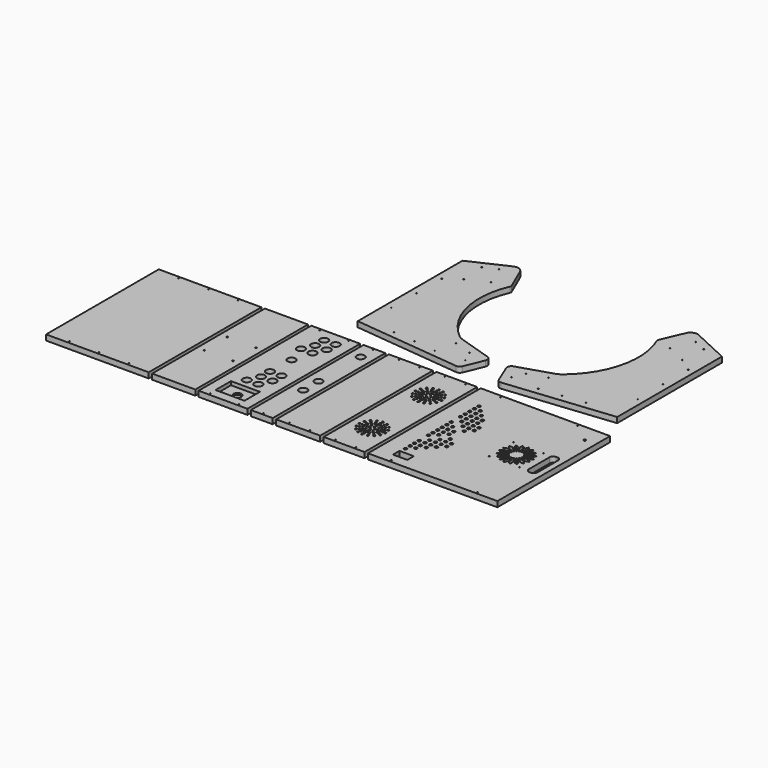
from build123d import *

# Parameters (mm, degrees)
F0_W      = 16
F0_H      = 420.523803
F0_R      = 14
F0_R_2    = 1.6
F1_DEPTH  = 19.05
F2_DEPTH  = 19.05
F0_W_2    = 357
F0_H_2    = 490
F3_DEPTH  = 19.05
F0_R_3    = 2.5
F4_DEPTH  = 19.05
F0_W_3    = 170
F0_W_4    = 98
F0_H_3    = 66
F5_DEPTH  = 19.05
F0_W_5    = 153
F6_DEPTH  = 19.05
F0_W_6    = 76
F7_DEPTH  = 19.05
F0_W_7    = 142
F0_R_4    = 3
F8_DEPTH  = 19.05
F0_W_8    = 450
F0_W_9    = 49.9710738659
F0_H_4    = 28.1445980072
F0_R_5    = 5
F0_R_6    = 1.75
F0_R_7    = 4
F9_DEPTH  = 19.05
F10_W     = 100.751042366
F10_H     = 67.1674013138
F10_R     = 14
F11_DEPTH = 12.7


# Not quite as in the source:
# - ends of sketch curves that miss each other by under 0.0002 mm in the source are joined
# - the dataset's text gives a spline's control points without its knots; the knots are read off the source's solid


with BuildPart() as f1:
    # F0 (on Top) → F1 (new body)
    with BuildSketch(Plane.XY):
        with BuildLine():
            ThreePointArc((118.5482367504, 140.3838887016), (29.2680787824, 284.7869007763), (44.0792440047, 453.913497998))
            ThreePointArc((44.0792440047, 453.913497998), (44.6945754076, 456.8856380721), (44.0816068861, 459.8582663821))
            Line((44.0816068861, 459.8582663821), (10.171633, 538.500267))
            ThreePointArc((10.171633, 538.500267), (-3.8765949653, 551.9603339279), (-23.3202071387, 551.2732802984))
            Line((-23.3202071387, 551.2732802984), (-152.1134, 491.42611))
            Line((-152.1134, 491.42611), (-152.1134, 35.994447))
            Line((-152.1134, 35.994447), (220.668635, -2.682718))
            ThreePointArc((220.668635, -2.682718), (229.9119854484, -0.638415896), (236.0902296243, 6.5343101544))
            Line((236.0902296243, 6.5343101544), (263.285491, 72.693217))
            ThreePointArc((263.285491, 72.693217), (263.0041902378, 84.740313744), (253.9506129321, 92.6929487862))
            Line((253.9506129321, 92.6929487862), (138.885599, 129.221951))
            ThreePointArc((138.885599, 129.221951), (128.172308682, 133.81062664), (118.5482367504, 140.3838887016))
        make_face()
        with Locations((-129.1134, 263.2859435)):
            Rectangle(F0_W, F0_H, mode=Mode.SUBTRACT)
        Polygon((20.257829, 446.91905), (-106.753851, 387.899707), (-113.091563, 402.597754), (13.920117, 461.617097), align=None, mode=Mode.SUBTRACT)
        Polygon((-11.034626, 519.490656), (-112.233483, 472.465925), (-118.975929, 486.975902), (-17.372338, 534.188703), align=None, mode=Mode.SUBTRACT)
        Polygon((196.938753, 31.951096), (195.287572, 16.036524), (-112.166792, 47.935762), (-110.515612, 63.850334), align=None, mode=Mode.SUBTRACT)
        with Locations((174.758149, 57.146597)):
            Circle(F0_R, mode=Mode.SUBTRACT)
        Polygon((96.986505, 104.752845), (103.090393, 119.601996), (241.766108, 75.577446), (235.66222, 60.728295), align=None, mode=Mode.SUBTRACT)
        Polygon((203.468062, 21.862117), (220.744217, 63.89045), (235.0899798126, 59.3361864098), (217.341675, 16.159233), align=None, mode=Mode.SUBTRACT)
        with Locations((-129.1134, 263.2859435)):
            Rectangle(F0_W, F0_H)
        with Locations((-129.6134, 153.285944)):
            Circle(F0_R_2, mode=Mode.SUBTRACT)
        with Locations((-129.6134, 263.285944)):
            Circle(F0_R_2, mode=Mode.SUBTRACT)
        with Locations((-129.6134, 373.285944)):
            Circle(F0_R_2, mode=Mode.SUBTRACT)
        Polygon((-113.091563, 402.597754), (-106.753851, 387.899707), (20.257829, 446.91905), (13.920117, 461.617097), align=None)
        with Locations((-80.973898, 408.376093)):
            Circle(F0_R_2, mode=Mode.SUBTRACT)
        with Locations((-11.54993, 440.408904)):
            Circle(F0_R_2, mode=Mode.SUBTRACT)
        Polygon((-118.975929, 486.975902), (-112.233483, 472.465925), (-11.034626, 519.490656), (-17.372338, 534.188703), align=None)
        with Locations((-87.024666, 493.674259)):
            Circle(F0_R_2, mode=Mode.SUBTRACT)
        with Locations((-43.238492, 513.899138)):
            Circle(F0_R_2, mode=Mode.SUBTRACT)
        Polygon((235.0899798126, 59.3361864098), (220.744217, 63.89045), (203.468062, 21.862117), (217.341675, 16.159233), align=None)
        with Locations((219.042946, 40.024842)):
            Circle(F0_R_2, mode=Mode.SUBTRACT)
        Polygon((241.766108, 75.577446), (103.090393, 119.601996), (96.986505, 104.752845), (235.66222, 60.728295), align=None)
        with Locations((138.165875, 100.597925)):
            Circle(F0_R_2, mode=Mode.SUBTRACT)
        with Locations((200.978281, 80.69215)):
            Circle(F0_R_2, mode=Mode.SUBTRACT)
        with Locations((174.758149, 57.146597)):
            Circle(F0_R)
        Polygon((-112.166792, 47.935762), (195.287572, 16.036524), (196.938753, 31.951096), (-110.515612, 63.850334), align=None)
        with Locations((-34.52921, 47.420908)):
            Circle(F0_R_2, mode=Mode.SUBTRACT)
        with Locations((42.334381, 39.446099)):
            Circle(F0_R_2, mode=Mode.SUBTRACT)
        with Locations((119.215626, 31.64332)):
            Circle(F0_R_2, mode=Mode.SUBTRACT)
    extrude(amount=F1_DEPTH)


with BuildPart() as f2:
    # F0 (on Top) → F2 (new body)
    with BuildSketch(Plane.XY):
        with BuildLine():
            Line((588.126429, 538.500267), (554.216456, 459.858266))
            ThreePointArc((554.216456, 459.858266), (553.6034865924, 456.8856380721), (554.2188179042, 453.9134979586))
            ThreePointArc((554.2188179042, 453.9134979586), (569.0299832176, 284.7869007763), (479.7498252496, 140.3838887016))
            ThreePointArc((479.7498252496, 140.3838887016), (470.125753318, 133.81062664), (459.4124630169, 129.2219509467))
            Line((459.4124630169, 129.2219509467), (344.347449, 92.692949))
            ThreePointArc((344.347449, 92.692949), (335.2938717622, 84.740313744), (335.0125713757, 72.6932171544))
            Line((335.0125713757, 72.6932171544), (362.207832, 6.53431))
            ThreePointArc((362.207832, 6.53431), (368.3860765516, -0.638415896), (377.6294270257, -2.682718248))
            Line((377.6294270257, -2.682718248), (750.411462, 35.994447))
            Line((750.411462, 35.994447), (750.411462, 491.42611))
            Line((750.411462, 491.42611), (621.618269, 551.27328))
            ThreePointArc((621.618269, 551.27328), (602.1746569653, 551.9603339279), (588.126429, 538.500267))
        make_face()
        Polygon((363.2080821874, 59.3361864098), (377.553845, 63.89045), (394.83, 21.862117), (380.956387, 16.159233), align=None, mode=Mode.SUBTRACT)
        with Locations((423.539913, 57.146597)):
            Circle(F0_R, mode=Mode.SUBTRACT)
        Polygon((710.464854, 47.935762), (403.01049, 16.036524), (401.359309, 31.951096), (708.813674, 63.850334), align=None, mode=Mode.SUBTRACT)
        Polygon((356.531954, 75.577446), (495.207669, 119.601996), (501.311557, 104.752845), (362.635842, 60.728295), align=None, mode=Mode.SUBTRACT)
        with Locations((727.411462, 263.2859435)):
            Rectangle(F0_W, F0_H, mode=Mode.SUBTRACT)
        Polygon((711.389625, 402.597754), (705.051913, 387.899707), (578.040233, 446.91905), (584.377945, 461.617097), align=None, mode=Mode.SUBTRACT)
        Polygon((717.273991, 486.975902), (710.531545, 472.465925), (609.332688, 519.490656), (615.6704, 534.188703), align=None, mode=Mode.SUBTRACT)
        Polygon((609.332688, 519.490656), (710.531545, 472.465925), (717.273991, 486.975902), (615.6704, 534.188703), align=None)
        with Locations((641.536554, 513.899138)):
            Circle(F0_R_2, mode=Mode.SUBTRACT)
        with Locations((685.322728, 493.674259)):
            Circle(F0_R_2, mode=Mode.SUBTRACT)
        Polygon((578.040233, 446.91905), (705.051913, 387.899707), (711.389625, 402.597754), (584.377945, 461.617097), align=None)
        with Locations((679.27196, 408.376093)):
            Circle(F0_R_2, mode=Mode.SUBTRACT)
        with Locations((609.847992, 440.408904)):
            Circle(F0_R_2, mode=Mode.SUBTRACT)
        with Locations((727.411462, 263.2859435)):
            Rectangle(F0_W, F0_H)
        with Locations((727.911462, 153.285944)):
            Circle(F0_R_2, mode=Mode.SUBTRACT)
        with Locations((727.911462, 263.285944)):
            Circle(F0_R_2, mode=Mode.SUBTRACT)
        with Locations((727.911462, 373.285944)):
            Circle(F0_R_2, mode=Mode.SUBTRACT)
        Polygon((501.311557, 104.752845), (495.207669, 119.601996), (356.531954, 75.577446), (362.635842, 60.728295), align=None)
        with Locations((397.319781, 80.69215)):
            Circle(F0_R_2, mode=Mode.SUBTRACT)
        with Locations((460.132187, 100.597925)):
            Circle(F0_R_2, mode=Mode.SUBTRACT)
        with Locations((423.539913, 57.146597)):
            Circle(F0_R)
        Polygon((394.83, 21.862117), (377.553845, 63.89045), (363.2080821874, 59.3361864098), (380.956387, 16.159233), align=None)
        with Locations((379.255116, 40.024842)):
            Circle(F0_R_2, mode=Mode.SUBTRACT)
        Polygon((401.359309, 31.951096), (403.01049, 16.036524), (710.464854, 47.935762), (708.813674, 63.850334), align=None)
        with Locations((479.082436, 31.64332)):
            Circle(F0_R_2, mode=Mode.SUBTRACT)
        with Locations((555.963681, 39.446099)):
            Circle(F0_R_2, mode=Mode.SUBTRACT)
        with Locations((632.827272, 47.420908)):
            Circle(F0_R_2, mode=Mode.SUBTRACT)
    extrude(amount=F2_DEPTH)


with BuildPart() as f3:
    # F0 (on Top) → F3 (new body)
    with BuildSketch(Plane.XY):
        with Locations((-586.06424, -308.60144)):
            Rectangle(F0_W_2, F0_H_2)
        with Locations((-689.56424, -546.10144)):
            Circle(F0_R_2, mode=Mode.SUBTRACT)
        with Locations((-586.06424, -546.10144)):
            Circle(F0_R_2, mode=Mode.SUBTRACT)
        with Locations((-482.56424, -546.10144)):
            Circle(F0_R_2, mode=Mode.SUBTRACT)
        with Locations((-689.56424, -71.10144)):
            Circle(F0_R_2, mode=Mode.SUBTRACT)
        with Locations((-586.06424, -71.10144)):
            Circle(F0_R_2, mode=Mode.SUBTRACT)
        with Locations((-482.56424, -71.10144)):
            Circle(F0_R_2, mode=Mode.SUBTRACT)
    extrude(amount=F3_DEPTH)


with BuildPart() as f4:
    # F0 (on Top) → F4 (new body)
    with BuildSketch(Plane.XY):
        Polygon((-395.373191, -518.60144), (-395.373191, -533.60144), (-395.373191, -553.60144), (-245.373191, -553.60144), (-245.373191, -533.60144), (-245.373191, -518.60144), (-245.373191, -98.60144), (-245.373191, -83.60144), (-245.373191, -63.60144), (-395.373191, -63.60144), align=None)
        with Locations((-370.373191, -358.60144)):
            Circle(F0_R_3, mode=Mode.SUBTRACT)
        with Locations((-270.373191, -358.60144)):
            Circle(F0_R_3, mode=Mode.SUBTRACT)
        with Locations((-370.373191, -258.60144)):
            Circle(F0_R_3, mode=Mode.SUBTRACT)
        with Locations((-270.373191, -258.60144)):
            Circle(F0_R_3, mode=Mode.SUBTRACT)
    extrude(amount=F4_DEPTH)


with BuildPart() as f5:
    # F0 (on Top) → F5 (new body)
    with BuildSketch(Plane.XY):
        with Locations((-149.025639, -308.60144)):
            Rectangle(F0_W_3, F0_H_2)
        with Locations((-199.025639, -546.60144)):
            Circle(F0_R_2, mode=Mode.SUBTRACT)
        with Locations((-99.025639, -546.60144)):
            Circle(F0_R_2, mode=Mode.SUBTRACT)
        with Locations((-150.025639, -489.60144)):
            Rectangle(F0_W_4, F0_H_3, mode=Mode.SUBTRACT)
        with Locations((-171.025639, -422.60144)):
            Circle(F0_R, mode=Mode.SUBTRACT)
        with Locations((-131.025639, -422.60144)):
            Circle(F0_R, mode=Mode.SUBTRACT)
        with Locations((-153.025639, -383.35144)):
            Circle(F0_R, mode=Mode.SUBTRACT)
        with Locations((-113.025639, -383.35144)):
            Circle(F0_R, mode=Mode.SUBTRACT)
        with Locations((-153.025639, -344.10144)):
            Circle(F0_R, mode=Mode.SUBTRACT)
        with Locations((-113.025639, -344.10144)):
            Circle(F0_R, mode=Mode.SUBTRACT)
        with Locations((-150.025639, -254.35144)):
            Rectangle(F0_W_4, F0_H_3, mode=Mode.SUBTRACT)
        with Locations((-171.025639, -187.35144)):
            Circle(F0_R, mode=Mode.SUBTRACT)
        with Locations((-131.025639, -187.35144)):
            Circle(F0_R, mode=Mode.SUBTRACT)
        with Locations((-153.025639, -148.10144)):
            Circle(F0_R, mode=Mode.SUBTRACT)
        with Locations((-113.025639, -148.10144)):
            Circle(F0_R, mode=Mode.SUBTRACT)
        with Locations((-199.025639, -70.60144)):
            Circle(F0_R_2, mode=Mode.SUBTRACT)
        with Locations((-153.025639, -108.85144)):
            Circle(F0_R, mode=Mode.SUBTRACT)
        with Locations((-113.025639, -108.85144)):
            Circle(F0_R, mode=Mode.SUBTRACT)
        with Locations((-99.025639, -70.60144)):
            Circle(F0_R_2, mode=Mode.SUBTRACT)
        with Locations((-150.025639, -254.35144)):
            Rectangle(F0_W_4, F0_H_3)
        with Locations((-150.025639, -254.35144)):
            Circle(F0_R, mode=Mode.SUBTRACT)
        with Locations((-150.025639, -489.60144)):
            Rectangle(F0_W_4, F0_H_3)
        with Locations((-150.025639, -489.60144)):
            Circle(F0_R, mode=Mode.SUBTRACT)
    extrude(amount=F5_DEPTH)

    # F10 (on face) → F11 (cut)
    with BuildSketch(Plane.XY.offset(19.05)):
        with Locations((-150.2750962973, -488.087952137)):
            Rectangle(F10_W, F10_H)
        with Locations((-150.025639, -489.60144)):
            Circle(F10_R, mode=Mode.SUBTRACT)
    extrude(amount=-F11_DEPTH, mode=Mode.SUBTRACT)


with BuildPart() as f6:
    # F0 (on Top) → F6 (new body)
    with BuildSketch(Plane.XY):
        with Locations((112.484238, -308.60144)):
            Rectangle(F0_W_5, F0_H_2)
        with Locations((76.484238, -546.60144)):
            Circle(F0_R_2, mode=Mode.SUBTRACT)
        with Locations((148.484238, -546.60144)):
            Circle(F0_R_2, mode=Mode.SUBTRACT)
        with Locations((76.484238, -70.60144)):
            Circle(F0_R_2, mode=Mode.SUBTRACT)
        with Locations((148.484238, -70.60144)):
            Circle(F0_R_2, mode=Mode.SUBTRACT)
    extrude(amount=F6_DEPTH)


with BuildPart() as f7:
    # F0 (on Top) → F7 (new body)
    with BuildSketch(Plane.XY):
        with Locations((-14.20681, -308.60144)):
            Rectangle(F0_W_6, F0_H_2)
        with Locations((-14.20681, -546.60144)):
            Circle(F0_R_2, mode=Mode.SUBTRACT)
        with Locations((-14.20681, -373.60144)):
            Circle(F0_R, mode=Mode.SUBTRACT)
        with Locations((-14.20681, -306.99525)):
            Circle(F0_R, mode=Mode.SUBTRACT)
        with Locations((-14.20681, -123.560914)):
            Circle(F0_R, mode=Mode.SUBTRACT)
        with Locations((-14.20681, -70.60144)):
            Circle(F0_R_2, mode=Mode.SUBTRACT)
    extrude(amount=F7_DEPTH)


with BuildPart() as f8:
    # F0 (on Top) → F8 (new body)
    with BuildSketch(Plane.XY):
        with Locations((272.175287, -308.60144)):
            Rectangle(F0_W_7, F0_H_2)
        with Locations((236.175287, -546.60144)):
            Circle(F0_R_2, mode=Mode.SUBTRACT)
        with Locations((308.175287, -546.60144)):
            Circle(F0_R_2, mode=Mode.SUBTRACT)
        with Locations((254.954532, -472.176019)):
            Circle(F0_R_4, mode=Mode.SUBTRACT)
        with Locations((240.355481, -462.421245)):
            Circle(F0_R_4, mode=Mode.SUBTRACT)
        with Locations((258.398683, -463.861103)):
            Circle(F0_R_4, mode=Mode.SUBTRACT)
        with Locations((246.719442, -456.057284)):
            Circle(F0_R_4, mode=Mode.SUBTRACT)
        with Locations((261.842834, -455.546188)):
            Circle(F0_R_4, mode=Mode.SUBTRACT)
        with Locations((272.175287, -475.60144)):
            Circle(F0_R_4, mode=Mode.SUBTRACT)
        with Locations((289.396041, -472.176019)):
            Circle(F0_R_4, mode=Mode.SUBTRACT)
        with Locations((272.175287, -466.60144)):
            Circle(F0_R_4, mode=Mode.SUBTRACT)
        with Locations((285.95189, -463.861103)):
            Circle(F0_R_4, mode=Mode.SUBTRACT)
        with Locations((272.175287, -457.60144)):
            Circle(F0_R_4, mode=Mode.SUBTRACT)
        with Locations((282.507739, -455.546188)):
            Circle(F0_R_4, mode=Mode.SUBTRACT)
        with Locations((303.995092, -462.421245)):
            Circle(F0_R_4, mode=Mode.SUBTRACT)
        with Locations((297.631131, -456.057284)):
            Circle(F0_R_4, mode=Mode.SUBTRACT)
        with Locations((230.600708, -447.822195)):
            Circle(F0_R_4, mode=Mode.SUBTRACT)
        with Locations((238.915623, -444.378044)):
            Circle(F0_R_4, mode=Mode.SUBTRACT)
        with Locations((253.083403, -449.693323)):
            Circle(F0_R_4, mode=Mode.SUBTRACT)
        with Locations((259.447364, -443.329362)):
            Circle(F0_R_4, mode=Mode.SUBTRACT)
        with Locations((247.230539, -440.933893)):
            Circle(F0_R_4, mode=Mode.SUBTRACT)
        with Locations((227.175287, -430.60144)):
            Circle(F0_R_4, mode=Mode.SUBTRACT)
        with Locations((236.175287, -430.60144)):
            Circle(F0_R_4, mode=Mode.SUBTRACT)
        with Locations((238.915623, -416.824837)):
            Circle(F0_R_4, mode=Mode.SUBTRACT)
        with Locations((245.175287, -430.60144)):
            Circle(F0_R_4, mode=Mode.SUBTRACT)
        with Locations((254.175287, -430.60144)):
            Circle(F0_R_4, mode=Mode.SUBTRACT)
        with Locations((263.175287, -430.60144)):
            Circle(F0_R_4, mode=Mode.SUBTRACT)
        with Locations((247.230539, -420.268988)):
            Circle(F0_R_4, mode=Mode.SUBTRACT)
        with Locations((259.447364, -417.873518)):
            Circle(F0_R_4, mode=Mode.SUBTRACT)
        with Locations((272.175287, -448.60144)):
            Circle(F0_R_4, mode=Mode.SUBTRACT)
        with Locations((284.903209, -443.329362)):
            Circle(F0_R_4, mode=Mode.SUBTRACT)
        with Locations((272.175287, -439.60144)):
            Circle(F0_R_4, mode=Mode.SUBTRACT)
        with Locations((291.26717, -449.693323)):
            Circle(F0_R_4, mode=Mode.SUBTRACT)
        with Locations((313.749866, -447.822195)):
            Circle(F0_R_4, mode=Mode.SUBTRACT)
        with Locations((305.43495, -444.378044)):
            Circle(F0_R_4, mode=Mode.SUBTRACT)
        with Locations((297.120034, -440.933893)):
            Circle(F0_R_4, mode=Mode.SUBTRACT)
        with Locations((281.175287, -430.60144)):
            Circle(F0_R_4, mode=Mode.SUBTRACT)
        with Locations((290.175287, -430.60144)):
            Circle(F0_R_4, mode=Mode.SUBTRACT)
        with Locations((272.175287, -421.60144)):
            Circle(F0_R_4, mode=Mode.SUBTRACT)
        with Locations((284.903209, -417.873518)):
            Circle(F0_R_4, mode=Mode.SUBTRACT)
        with Locations((299.175287, -430.60144)):
            Circle(F0_R_4, mode=Mode.SUBTRACT)
        with Locations((308.175287, -430.60144)):
            Circle(F0_R_4, mode=Mode.SUBTRACT)
        with Locations((297.120034, -420.268988)):
            Circle(F0_R_4, mode=Mode.SUBTRACT)
        with Locations((305.43495, -416.824837)):
            Circle(F0_R_4, mode=Mode.SUBTRACT)
        with Locations((317.175287, -430.60144)):
            Circle(F0_R_4, mode=Mode.SUBTRACT)
        with Locations((230.600708, -413.380686)):
            Circle(F0_R_4, mode=Mode.SUBTRACT)
        with Locations((240.355481, -398.781635)):
            Circle(F0_R_4, mode=Mode.SUBTRACT)
        with Locations((253.083403, -411.509557)):
            Circle(F0_R_4, mode=Mode.SUBTRACT)
        with Locations((246.719442, -405.145596)):
            Circle(F0_R_4, mode=Mode.SUBTRACT)
        with Locations((261.842834, -405.656693)):
            Circle(F0_R_4, mode=Mode.SUBTRACT)
        with Locations((258.398683, -397.341777)):
            Circle(F0_R_4, mode=Mode.SUBTRACT)
        with Locations((254.954532, -389.026861)):
            Circle(F0_R_4, mode=Mode.SUBTRACT)
        with Locations((272.175287, -412.60144)):
            Circle(F0_R_4, mode=Mode.SUBTRACT)
        with Locations((272.175287, -403.60144)):
            Circle(F0_R_4, mode=Mode.SUBTRACT)
        with Locations((282.507739, -405.656693)):
            Circle(F0_R_4, mode=Mode.SUBTRACT)
        with Locations((291.26717, -411.509557)):
            Circle(F0_R_4, mode=Mode.SUBTRACT)
        with Locations((313.749866, -413.380686)):
            Circle(F0_R_4, mode=Mode.SUBTRACT)
        with Locations((297.631131, -405.145596)):
            Circle(F0_R_4, mode=Mode.SUBTRACT)
        with Locations((303.995092, -398.781635)):
            Circle(F0_R_4, mode=Mode.SUBTRACT)
        with Locations((272.175287, -394.60144)):
            Circle(F0_R_4, mode=Mode.SUBTRACT)
        with Locations((285.95189, -397.341777)):
            Circle(F0_R_4, mode=Mode.SUBTRACT)
        with Locations((272.175287, -385.60144)):
            Circle(F0_R_4, mode=Mode.SUBTRACT)
        with Locations((289.396041, -389.026861)):
            Circle(F0_R_4, mode=Mode.SUBTRACT)
        with Locations((254.954532, -228.176019)):
            Circle(F0_R_4, mode=Mode.SUBTRACT)
        with Locations((240.355481, -218.421245)):
            Circle(F0_R_4, mode=Mode.SUBTRACT)
        with Locations((258.398683, -219.861103)):
            Circle(F0_R_4, mode=Mode.SUBTRACT)
        with Locations((246.719442, -212.057284)):
            Circle(F0_R_4, mode=Mode.SUBTRACT)
        with Locations((261.842834, -211.546188)):
            Circle(F0_R_4, mode=Mode.SUBTRACT)
        with Locations((272.175287, -231.60144)):
            Circle(F0_R_4, mode=Mode.SUBTRACT)
        with Locations((289.396041, -228.176019)):
            Circle(F0_R_4, mode=Mode.SUBTRACT)
        with Locations((272.175287, -222.60144)):
            Circle(F0_R_4, mode=Mode.SUBTRACT)
        with Locations((285.95189, -219.861103)):
            Circle(F0_R_4, mode=Mode.SUBTRACT)
        with Locations((272.175287, -213.60144)):
            Circle(F0_R_4, mode=Mode.SUBTRACT)
        with Locations((282.507739, -211.546188)):
            Circle(F0_R_4, mode=Mode.SUBTRACT)
        with Locations((303.995092, -218.421245)):
            Circle(F0_R_4, mode=Mode.SUBTRACT)
        with Locations((297.631131, -212.057284)):
            Circle(F0_R_4, mode=Mode.SUBTRACT)
        with Locations((230.600708, -203.822195)):
            Circle(F0_R_4, mode=Mode.SUBTRACT)
        with Locations((238.915623, -200.378044)):
            Circle(F0_R_4, mode=Mode.SUBTRACT)
        with Locations((253.083403, -205.693323)):
            Circle(F0_R_4, mode=Mode.SUBTRACT)
        with Locations((259.447364, -199.329362)):
            Circle(F0_R_4, mode=Mode.SUBTRACT)
        with Locations((247.230539, -196.933893)):
            Circle(F0_R_4, mode=Mode.SUBTRACT)
        with Locations((227.175287, -186.60144)):
            Circle(F0_R_4, mode=Mode.SUBTRACT)
        with Locations((236.175287, -186.60144)):
            Circle(F0_R_4, mode=Mode.SUBTRACT)
        with Locations((245.175287, -186.60144)):
            Circle(F0_R_4, mode=Mode.SUBTRACT)
        with Locations((254.175287, -186.60144)):
            Circle(F0_R_4, mode=Mode.SUBTRACT)
        with Locations((263.175287, -186.60144)):
            Circle(F0_R_4, mode=Mode.SUBTRACT)
        with Locations((247.230539, -176.268988)):
            Circle(F0_R_4, mode=Mode.SUBTRACT)
        with Locations((259.447364, -173.873518)):
            Circle(F0_R_4, mode=Mode.SUBTRACT)
        with Locations((272.175287, -204.60144)):
            Circle(F0_R_4, mode=Mode.SUBTRACT)
        with Locations((284.903209, -199.329362)):
            Circle(F0_R_4, mode=Mode.SUBTRACT)
        with Locations((272.175287, -195.60144)):
            Circle(F0_R_4, mode=Mode.SUBTRACT)
        with Locations((291.26717, -205.693323)):
            Circle(F0_R_4, mode=Mode.SUBTRACT)
        with Locations((313.749866, -203.822195)):
            Circle(F0_R_4, mode=Mode.SUBTRACT)
        with Locations((305.43495, -200.378044)):
            Circle(F0_R_4, mode=Mode.SUBTRACT)
        with Locations((297.120034, -196.933893)):
            Circle(F0_R_4, mode=Mode.SUBTRACT)
        with Locations((281.175287, -186.60144)):
            Circle(F0_R_4, mode=Mode.SUBTRACT)
        with Locations((290.175287, -186.60144)):
            Circle(F0_R_4, mode=Mode.SUBTRACT)
        with Locations((272.175287, -177.60144)):
            Circle(F0_R_4, mode=Mode.SUBTRACT)
        with Locations((284.903209, -173.873518)):
            Circle(F0_R_4, mode=Mode.SUBTRACT)
        with Locations((299.175287, -186.60144)):
            Circle(F0_R_4, mode=Mode.SUBTRACT)
        with Locations((308.175287, -186.60144)):
            Circle(F0_R_4, mode=Mode.SUBTRACT)
        with Locations((297.120034, -176.268988)):
            Circle(F0_R_4, mode=Mode.SUBTRACT)
        with Locations((230.600708, -169.380686)):
            Circle(F0_R_4, mode=Mode.SUBTRACT)
        with Locations((238.915623, -172.824837)):
            Circle(F0_R_4, mode=Mode.SUBTRACT)
        with Locations((253.083403, -167.509557)):
            Circle(F0_R_4, mode=Mode.SUBTRACT)
        with Locations((246.719442, -161.145596)):
            Circle(F0_R_4, mode=Mode.SUBTRACT)
        with Locations((261.842834, -161.656693)):
            Circle(F0_R_4, mode=Mode.SUBTRACT)
        with Locations((240.355481, -154.781635)):
            Circle(F0_R_4, mode=Mode.SUBTRACT)
        with Locations((258.398683, -153.341777)):
            Circle(F0_R_4, mode=Mode.SUBTRACT)
        with Locations((254.954532, -145.026861)):
            Circle(F0_R_4, mode=Mode.SUBTRACT)
        with Locations((272.175287, -168.60144)):
            Circle(F0_R_4, mode=Mode.SUBTRACT)
        with Locations((272.175287, -159.60144)):
            Circle(F0_R_4, mode=Mode.SUBTRACT)
        with Locations((282.507739, -161.656693)):
            Circle(F0_R_4, mode=Mode.SUBTRACT)
        with Locations((291.26717, -167.509557)):
            Circle(F0_R_4, mode=Mode.SUBTRACT)
        with Locations((305.43495, -172.824837)):
            Circle(F0_R_4, mode=Mode.SUBTRACT)
        with Locations((313.749866, -169.380686)):
            Circle(F0_R_4, mode=Mode.SUBTRACT)
        with Locations((297.631131, -161.145596)):
            Circle(F0_R_4, mode=Mode.SUBTRACT)
        with Locations((272.175287, -150.60144)):
            Circle(F0_R_4, mode=Mode.SUBTRACT)
        with Locations((285.95189, -153.341777)):
            Circle(F0_R_4, mode=Mode.SUBTRACT)
        with Locations((272.175287, -141.60144)):
            Circle(F0_R_4, mode=Mode.SUBTRACT)
        with Locations((289.396041, -145.026861)):
            Circle(F0_R_4, mode=Mode.SUBTRACT)
        with Locations((303.995092, -154.781635)):
            Circle(F0_R_4, mode=Mode.SUBTRACT)
        with Locations((317.175287, -186.60144)):
            Circle(F0_R_4, mode=Mode.SUBTRACT)
        with Locations((236.175287, -70.60144)):
            Circle(F0_R_2, mode=Mode.SUBTRACT)
        with Locations((308.175287, -70.60144)):
            Circle(F0_R_2, mode=Mode.SUBTRACT)
    extrude(amount=F8_DEPTH)


with BuildPart() as f9:
    # F0 (on Top) → F9 (new body)
    with BuildSketch(Plane.XY):
        with Locations((580.366335, -308.60144)):
            Rectangle(F0_W_8, F0_H_2)
        with Locations((430.366335, -546.10144)):
            Circle(F0_R_2, mode=Mode.SUBTRACT)
        with Locations((438.1191283464, -503.1597018242)):
            Rectangle(F0_W_9, F0_H_4, mode=Mode.SUBTRACT)
        with Locations((417.50945, -468.60144)):
            Circle(F0_R_5, mode=Mode.SUBTRACT)
        with Locations((417.50945, -448.60144)):
            Circle(F0_R_5, mode=Mode.SUBTRACT)
        with Locations((437.50945, -448.60144)):
            Circle(F0_R_5, mode=Mode.SUBTRACT)
        with Locations((417.50945, -428.60144)):
            Circle(F0_R_5, mode=Mode.SUBTRACT)
        with Locations((437.50945, -428.60144)):
            Circle(F0_R_5, mode=Mode.SUBTRACT)
        with Locations((457.50945, -428.60144)):
            Circle(F0_R_5, mode=Mode.SUBTRACT)
        with Locations((730.366335, -546.10144)):
            Circle(F0_R_2, mode=Mode.SUBTRACT)
        with Locations((417.50945, -408.60144)):
            Circle(F0_R_5, mode=Mode.SUBTRACT)
        with Locations((437.50945, -408.60144)):
            Circle(F0_R_5, mode=Mode.SUBTRACT)
        with Locations((457.50945, -408.60144)):
            Circle(F0_R_5, mode=Mode.SUBTRACT)
        with Locations((437.50945, -388.60144)):
            Circle(F0_R_5, mode=Mode.SUBTRACT)
        with Locations((457.50945, -388.60144)):
            Circle(F0_R_5, mode=Mode.SUBTRACT)
        with Locations((477.50945, -408.60144)):
            Circle(F0_R_5, mode=Mode.SUBTRACT)
        with Locations((477.50945, -388.60144)):
            Circle(F0_R_5, mode=Mode.SUBTRACT)
        with Locations((497.50945, -388.60144)):
            Circle(F0_R_5, mode=Mode.SUBTRACT)
        with Locations((417.50945, -368.60144)):
            Circle(F0_R_5, mode=Mode.SUBTRACT)
        with Locations((457.50945, -368.60144)):
            Circle(F0_R_5, mode=Mode.SUBTRACT)
        with Locations((417.50945, -348.60144)):
            Circle(F0_R_5, mode=Mode.SUBTRACT)
        with Locations((437.50945, -348.60144)):
            Circle(F0_R_5, mode=Mode.SUBTRACT)
        with Locations((477.50945, -368.60144)):
            Circle(F0_R_5, mode=Mode.SUBTRACT)
        with Locations((497.50945, -368.60144)):
            Circle(F0_R_5, mode=Mode.SUBTRACT)
        with Locations((477.50945, -348.60144)):
            Circle(F0_R_5, mode=Mode.SUBTRACT)
        with Locations((417.50945, -328.60144)):
            Circle(F0_R_5, mode=Mode.SUBTRACT)
        with Locations((437.50945, -328.60144)):
            Circle(F0_R_5, mode=Mode.SUBTRACT)
        with Locations((457.50945, -328.60144)):
            Circle(F0_R_5, mode=Mode.SUBTRACT)
        with Locations((417.50945, -308.60144)):
            Circle(F0_R_5, mode=Mode.SUBTRACT)
        with Locations((437.50945, -308.60144)):
            Circle(F0_R_5, mode=Mode.SUBTRACT)
        with Locations((457.50945, -308.60144)):
            Circle(F0_R_5, mode=Mode.SUBTRACT)
        with Locations((417.50945, -288.60144)):
            Circle(F0_R_5, mode=Mode.SUBTRACT)
        with Locations((437.50945, -288.60144)):
            Circle(F0_R_5, mode=Mode.SUBTRACT)
        with Locations((477.50945, -288.60144)):
            Circle(F0_R_5, mode=Mode.SUBTRACT)
        with Locations((623.107999, -361.10144)):
            Circle(F0_R_6, mode=Mode.SUBTRACT)
        with Locations((728.107999, -361.10144)):
            Circle(F0_R_6, mode=Mode.SUBTRACT)
        with BuildLine():
            add(Edge.make_bspline(
                [(661.9953345663, -323.6310243721), (662.2030436822, -323.6760680767), (664.8658202707, -324.6021810604), (656.014578, -335.388698), (653.296445, -345.742326), (644.42536, -349.015733), (640.039488, -350.634108)],
                knots=[37.385436, 37.385436, 37.385436, 37.385436, 38.16553, 48.738332, 61.900361, 74.770872, 74.770872, 74.770872, 74.770872], degree=3))
            add(Edge.make_bspline(
                [(640.039488, -350.634108), (640.014511, -346.232188), (639.95701, -336.098186), (653.509426, -332.830412), (655.8785976685, -324.3462786702), (660.5741339851, -323.3228234589), (661.9953345663, -323.6310243721)],
                knots=[0, 0, 0, 0, 12.01872, 27.669227, 32.047827, 37.385436, 37.385436, 37.385436, 37.385436], degree=3))
        make_face(mode=Mode.SUBTRACT)
        with BuildLine():
            add(Edge.make_bspline(
                [(657.6758589757, -318.0688243557), (657.8556358402, -318.1821923098), (660.041077992, -319.963177284), (648.034425, -327.071884), (641.939066, -335.871455), (632.483401, -335.913362), (627.808512, -335.934081)],
                knots=[37.385436, 37.385436, 37.385436, 37.385436, 38.16553, 48.738332, 61.900361, 74.770872, 74.770872, 74.770872, 74.770872], degree=3))
            add(Edge.make_bspline(
                [(627.808512, -335.934081), (629.290587, -331.789087), (632.702587, -322.246573), (646.555337, -323.811069), (651.6833751837, -316.648895877), (656.4457782291, -317.2931308976), (657.6758589757, -318.0688243557)],
                knots=[0, 0, 0, 0, 12.01872, 27.669227, 32.047827, 37.385436, 37.385436, 37.385436, 37.385436], degree=3))
        make_face(mode=Mode.SUBTRACT)
        with BuildLine():
            add(Edge.make_bspline(
                [(655.5192629717, -311.3647179179), (655.6494238634, -311.5327362358), (657.0939353029, -313.9537796275), (643.380051, -316.527262), (634.642656, -322.711419), (625.742905, -319.516771), (621.34286, -317.937334)],
                knots=[37.385436, 37.385436, 37.385436, 37.385436, 38.16553, 48.738332, 61.900361, 74.770872, 74.770872, 74.770872, 74.770872], degree=3))
            add(Edge.make_bspline(
                [(621.34286, -317.937334), (624.153227, -314.549213), (630.62319, -306.749156), (643.105427, -312.957221), (650.3738137707, -307.9808719712), (654.6286678035, -310.21509225), (655.5192629717, -311.3647179179)],
                knots=[0, 0, 0, 0, 12.01872, 27.669227, 32.047827, 37.385436, 37.385436, 37.385436, 37.385436], degree=3))
        make_face(mode=Mode.SUBTRACT)
        with BuildLine():
            add(Edge.make_bspline(
                [(667.9566993628, -327.3804345901), (668.1672879531, -327.3517211294), (670.9862289376, -327.311259493), (666.357988, -340.474573), (667.344928, -351.133457), (660.128406, -357.243543), (656.560551, -360.264375)],
                knots=[37.385436, 37.385436, 37.385436, 37.385436, 38.16553, 48.738332, 61.900361, 74.770872, 74.770872, 74.770872, 74.770872], degree=3))
            add(Edge.make_bspline(
                [(656.560551, -360.264375), (655.031535, -356.136466), (651.511469, -346.633286), (663.12893, -338.927383), (662.4534779475, -330.144600914), (666.5157966577, -327.5768996647), (667.9566993628, -327.3804345901)],
                knots=[0, 0, 0, 0, 12.01872, 27.669227, 32.047827, 37.385436, 37.385436, 37.385436, 37.385436], degree=3))
        make_face(mode=Mode.SUBTRACT)
        with BuildLine():
            add(Edge.make_bspline(
                [(674.8409233367, -328.8648210275), (675.02899128, -328.7658136803), (677.6640903625, -327.7636578564), (677.817085, -341.716078), (682.390058, -351.394599), (677.698518, -359.604398), (675.379017, -363.66333)],
                knots=[37.385436, 37.385436, 37.385436, 37.385436, 38.16553, 48.738332, 61.900361, 74.770872, 74.770872, 74.770872, 74.770872], degree=3))
            add(Edge.make_bspline(
                [(675.379017, -363.66333), (672.530384, -360.307318), (665.972325, -352.581183), (674.253593, -341.366598), (670.61498779, -333.344499859), (673.554112841, -329.542255423), (674.8409233367, -328.8648210275)],
                knots=[0, 0, 0, 0, 12.01872, 27.669227, 32.047827, 37.385436, 37.385436, 37.385436, 37.385436], degree=3))
        make_face(mode=Mode.SUBTRACT)
        with BuildLine():
            add(Edge.make_bspline(
                [(681.8176685037, -327.9051449566), (681.9605320608, -327.7477854641), (684.093957812, -325.904810145), (689.009734, -338.963469), (696.617172, -346.494255), (695.016484, -355.813544), (694.225102, -360.421008)],
                knots=[37.385436, 37.385436, 37.385436, 37.385436, 38.16553, 48.738332, 61.900361, 74.770872, 74.770872, 74.770872, 74.770872], degree=3))
            add(Edge.make_bspline(
                [(694.225102, -360.421008), (690.400439, -358.241679), (681.595385, -353.224475), (685.541618, -339.853851), (679.3787282548, -333.5600210155), (680.8401583471, -328.9818401281), (681.8176685037, -327.9051449566)],
                knots=[0, 0, 0, 0, 12.01872, 27.669227, 32.047827, 37.385436, 37.385436, 37.385436, 37.385436], degree=3))
        make_face(mode=Mode.SUBTRACT)
        with BuildLine():
            add(Edge.make_bspline(
                [(688.0454353909, -324.6171566724), (688.1258630897, -324.4204248936), (689.5002926346, -321.9589198656), (698.585936, -332.548751), (708.31027, -337.023478), (709.993499, -346.328213), (710.825689, -350.928482)],
                knots=[37.385436, 37.385436, 37.385436, 37.385436, 38.16553, 48.738332, 61.900361, 74.770872, 74.770872, 74.770872, 74.770872], degree=3))
            add(Edge.make_bspline(
                [(710.825689, -350.928482), (706.486307, -350.188693), (696.496278, -348.48557), (695.631501, -334.571603), (687.6876631469, -330.7651689726), (687.495127852, -325.963247417), (688.0454353909, -324.6171566724)],
                knots=[0, 0, 0, 0, 12.01872, 27.669227, 32.047827, 37.385436, 37.385436, 37.385436, 37.385436], degree=3))
        make_face(mode=Mode.SUBTRACT)
        with BuildLine():
            add(Edge.make_bspline(
                [(655.7856650626, -304.3273199728), (655.8505106214, -304.5297231889), (656.3798614587, -307.2988117366), (642.612843, -305.026669), (632.287272, -307.849511), (625.016875, -301.803629), (621.422385, -298.81454)],
                knots=[37.385436, 37.385436, 37.385436, 37.385436, 38.16553, 48.738332, 61.900361, 74.770872, 74.770872, 74.770872, 74.770872], degree=3))
            add(Edge.make_bspline(
                [(621.422385, -298.81454), (625.222071, -296.59195), (633.969624, -291.475152), (643.575807, -301.578001), (652.1078684137, -299.3876976547), (655.3419746379, -302.9424237577), (655.7856650626, -304.3273199728)],
                knots=[0, 0, 0, 0, 12.01872, 27.669227, 32.047827, 37.385436, 37.385436, 37.385436, 37.385436], degree=3))
        make_face(mode=Mode.SUBTRACT)
        with BuildLine():
            add(Edge.make_bspline(
                [(658.442933639, -297.8054433781), (658.4346425602, -298.0178186867), (657.9849856295, -300.8009596065), (645.825338, -293.957247), (635.157006, -293.078297), (630.392882, -284.910404), (628.037494, -280.872191)],
                knots=[37.385436, 37.385436, 37.385436, 37.385436, 38.16553, 48.738332, 61.900361, 74.770872, 74.770872, 74.770872, 74.770872], degree=3))
            add(Edge.make_bspline(
                [(628.037494, -280.872191), (632.368202, -280.083209), (642.338261, -278.26683), (647.909742, -291.045911), (656.6763853938, -291.905836018), (658.4996633881, -296.3523154746), (658.442933639, -297.8054433781)],
                knots=[0, 0, 0, 0, 12.01872, 27.669227, 32.047827, 37.385436, 37.385436, 37.385436, 37.385436], degree=3))
        make_face(mode=Mode.SUBTRACT)
        with BuildLine():
            add(Edge.make_bspline(
                [(663.1705620516, -292.5857233777), (663.090134334, -292.7824551636), (661.7157045442, -295.2439603132), (652.630062, -284.65413), (642.905727, -280.179402), (641.222498, -270.874668), (640.390308, -266.274399)],
                knots=[37.385436, 37.385436, 37.385436, 37.385436, 38.16553, 48.738332, 61.900361, 74.770872, 74.770872, 74.770872, 74.770872], degree=3))
            add(Edge.make_bspline(
                [(640.390308, -266.274399), (644.729691, -267.014187), (654.719719, -268.717311), (655.584496, -282.631278), (663.5283348232, -286.4377110572), (663.7208697189, -291.2396325852), (663.1705620516, -292.5857233777)],
                knots=[0, 0, 0, 0, 12.01872, 27.669227, 32.047827, 37.385436, 37.385436, 37.385436, 37.385436], degree=3))
        make_face(mode=Mode.SUBTRACT)
        with BuildLine():
            add(Edge.make_bspline(
                [(689.2206624337, -293.5718566276), (689.0129533178, -293.5268129233), (686.3501767293, -292.6006999396), (695.201419, -281.814183), (697.919552, -271.460555), (706.790637, -268.187148), (711.17651, -266.568772)],
                knots=[37.385436, 37.385436, 37.385436, 37.385436, 38.16553, 48.738332, 61.900361, 74.770872, 74.770872, 74.770872, 74.770872], degree=3))
            add(Edge.make_bspline(
                [(711.17651, -266.568772), (711.201486, -270.970692), (711.258987, -281.104694), (697.706571, -284.372468), (695.3373993315, -292.8566023), (690.6418630149, -293.8800575389), (689.2206624337, -293.5718566276)],
                knots=[0, 0, 0, 0, 12.01872, 27.669227, 32.047827, 37.385436, 37.385436, 37.385436, 37.385436], degree=3))
        make_face(mode=Mode.SUBTRACT)
        with BuildLine():
            add(Edge.make_bspline(
                [(692.773063361, -319.3974376216), (692.7813544398, -319.1850623133), (693.2310113705, -316.4019213935), (705.390659, -323.245634), (716.058991, -324.124584), (720.823116, -332.292476), (723.178503, -336.330689)],
                knots=[37.385436, 37.385436, 37.385436, 37.385436, 38.16553, 48.738332, 61.900361, 74.770872, 74.770872, 74.770872, 74.770872], degree=3))
            add(Edge.make_bspline(
                [(723.178503, -336.330689), (718.847795, -337.119672), (708.877736, -338.93605), (703.306255, -326.156969), (694.5396116062, -325.2970449521), (692.7163336119, -320.8505655232), (692.773063361, -319.3974376216)],
                knots=[0, 0, 0, 0, 12.01872, 27.669227, 32.047827, 37.385436, 37.385436, 37.385436, 37.385436], degree=3))
        make_face(mode=Mode.SUBTRACT)
        with BuildLine():
            add(Edge.make_bspline(
                [(695.4303319374, -312.8755609774), (695.3654863786, -312.6731577539), (694.8361355413, -309.9040690846), (708.603154, -312.176211), (718.928726, -309.35337), (726.199122, -315.399251), (729.793612, -318.38834)],
                knots=[37.385436, 37.385436, 37.385436, 37.385436, 38.16553, 48.738332, 61.900361, 74.770872, 74.770872, 74.770872, 74.770872], degree=3))
            add(Edge.make_bspline(
                [(729.793612, -318.38834), (725.993926, -320.610931), (717.246373, -325.727729), (707.64019, -315.62488), (699.1081285863, -317.8151833453), (695.8740223621, -314.2604572423), (695.4303319374, -312.8755609774)],
                knots=[0, 0, 0, 0, 12.01872, 27.669227, 32.047827, 37.385436, 37.385436, 37.385436, 37.385436], degree=3))
        make_face(mode=Mode.SUBTRACT)
        with BuildLine():
            add(Edge.make_bspline(
                [(695.6967346355, -305.8381624749), (695.5665737701, -305.6701441307), (694.1220626971, -303.2491003725), (707.835947, -300.675618), (716.573341, -294.491462), (725.473092, -297.68611), (729.873137, -299.265547)],
                knots=[37.385436, 37.385436, 37.385436, 37.385436, 38.16553, 48.738332, 61.900361, 74.770872, 74.770872, 74.770872, 74.770872], degree=3))
            add(Edge.make_bspline(
                [(729.873137, -299.265547), (727.06277, -302.653668), (720.592808, -310.453724), (708.11057, -304.24566), (700.8421832293, -309.2220090288), (696.5873296234, -306.9877883231), (695.6967346355, -305.8381624749)],
                knots=[0, 0, 0, 0, 12.01872, 27.669227, 32.047827, 37.385436, 37.385436, 37.385436, 37.385436], degree=3))
        make_face(mode=Mode.SUBTRACT)
        with BuildLine():
            add(Edge.make_bspline(
                [(693.5401390243, -299.1340562515), (693.3603621598, -299.0206883237), (691.174920008, -297.239703716), (703.181573, -290.130997), (709.276932, -281.331425), (718.732596, -281.289518), (723.407485, -281.268799)],
                knots=[37.385436, 37.385436, 37.385436, 37.385436, 38.16553, 48.738332, 61.900361, 74.770872, 74.770872, 74.770872, 74.770872], degree=3))
            add(Edge.make_bspline(
                [(723.407485, -281.268799), (721.92541, -285.413794), (718.51341, -294.956307), (704.660661, -293.391811), (699.5326228163, -300.553984123), (694.7702197709, -299.9097495293), (693.5401390243, -299.1340562515)],
                knots=[0, 0, 0, 0, 12.01872, 27.669227, 32.047827, 37.385436, 37.385436, 37.385436, 37.385436], degree=3))
        make_face(mode=Mode.SUBTRACT)
        with BuildLine():
            ThreePointArc((784.87855196, -353.6314878941), (781.1588080811, -362.6117440151), (772.17855196, -366.3314878941))
            Line((772.17855196, -366.3314878941), (767.5241019249, -366.3314878941))
            ThreePointArc((767.5241019249, -366.3314878941), (758.5438458038, -362.6117440151), (754.8241019249, -353.6314878941))
            Line((754.8241019249, -353.6314878941), (754.8241019249, -263.5713921059))
            ThreePointArc((754.8241019249, -263.5713921059), (758.5438458038, -254.5911359849), (767.5241019249, -250.8713921059))
            Line((767.5241019249, -250.8713921059), (772.17855196, -250.8713921059))
            ThreePointArc((772.17855196, -250.8713921059), (781.1588080811, -254.5911359849), (784.87855196, -263.5713921059))
            Line((784.87855196, -263.5713921059), (784.87855196, -353.6314878941))
        make_face(mode=Mode.SUBTRACT)
        with Locations((417.50945, -268.60144)):
            Circle(F0_R_5, mode=Mode.SUBTRACT)
        with Locations((457.50945, -268.60144)):
            Circle(F0_R_5, mode=Mode.SUBTRACT)
        with Locations((437.50945, -248.60144)):
            Circle(F0_R_5, mode=Mode.SUBTRACT)
        with Locations((457.50945, -248.60144)):
            Circle(F0_R_5, mode=Mode.SUBTRACT)
        with Locations((477.50945, -268.60144)):
            Circle(F0_R_5, mode=Mode.SUBTRACT)
        with Locations((497.50945, -268.60144)):
            Circle(F0_R_5, mode=Mode.SUBTRACT)
        with Locations((477.50945, -248.60144)):
            Circle(F0_R_5, mode=Mode.SUBTRACT)
        with Locations((497.50945, -248.60144)):
            Circle(F0_R_5, mode=Mode.SUBTRACT)
        with Locations((417.50945, -228.60144)):
            Circle(F0_R_5, mode=Mode.SUBTRACT)
        with Locations((437.50945, -228.60144)):
            Circle(F0_R_5, mode=Mode.SUBTRACT)
        with Locations((457.50945, -228.60144)):
            Circle(F0_R_5, mode=Mode.SUBTRACT)
        with Locations((417.50945, -208.60144)):
            Circle(F0_R_5, mode=Mode.SUBTRACT)
        with Locations((437.50945, -208.60144)):
            Circle(F0_R_5, mode=Mode.SUBTRACT)
        with Locations((457.50945, -208.60144)):
            Circle(F0_R_5, mode=Mode.SUBTRACT)
        with Locations((477.50945, -228.60144)):
            Circle(F0_R_5, mode=Mode.SUBTRACT)
        with Locations((477.50945, -208.60144)):
            Circle(F0_R_5, mode=Mode.SUBTRACT)
        with Locations((417.50945, -188.60144)):
            Circle(F0_R_5, mode=Mode.SUBTRACT)
        with Locations((437.50945, -188.60144)):
            Circle(F0_R_5, mode=Mode.SUBTRACT)
        with Locations((457.50945, -188.60144)):
            Circle(F0_R_5, mode=Mode.SUBTRACT)
        with Locations((417.50945, -168.60144)):
            Circle(F0_R_5, mode=Mode.SUBTRACT)
        with Locations((437.50945, -168.60144)):
            Circle(F0_R_5, mode=Mode.SUBTRACT)
        with Locations((417.50945, -148.60144)):
            Circle(F0_R_5, mode=Mode.SUBTRACT)
        with Locations((623.107999, -256.10144)):
            Circle(F0_R_6, mode=Mode.SUBTRACT)
        with BuildLine():
            add(Edge.make_bspline(
                [(669.3983294464, -289.2977356506), (669.255465882, -289.4550951694), (667.1220400092, -291.298070855), (662.206263, -278.239412), (654.598825, -270.708626), (656.199514, -261.389337), (656.990896, -256.781872)],
                knots=[37.385436, 37.385436, 37.385436, 37.385436, 38.16553, 48.738332, 61.900361, 74.770872, 74.770872, 74.770872, 74.770872], degree=3))
            add(Edge.make_bspline(
                [(656.990896, -256.781872), (660.815559, -258.961202), (669.620612, -263.978406), (665.67438, -277.349029), (671.8372697452, -283.6428589845), (670.3758396529, -288.2210402988), (669.3983294464, -289.2977356506)],
                knots=[0, 0, 0, 0, 12.01872, 27.669227, 32.047827, 37.385436, 37.385436, 37.385436, 37.385436], degree=3))
        make_face(mode=Mode.SUBTRACT)
        with BuildLine():
            add(Edge.make_bspline(
                [(676.3750736633, -288.3380595797), (676.18700572, -288.4370669532), (673.5519066375, -289.4392231436), (673.398912, -275.486803), (668.825939, -265.808281), (673.517479, -257.598482), (675.836981, -253.53955)],
                knots=[37.385436, 37.385436, 37.385436, 37.385436, 38.16553, 48.738332, 61.900361, 74.770872, 74.770872, 74.770872, 74.770872], degree=3))
            add(Edge.make_bspline(
                [(675.836981, -253.53955), (678.685614, -256.895562), (685.243673, -264.621697), (676.962404, -275.836282), (680.60100921, -283.858380141), (677.661884159, -287.6606250039), (676.3750736633, -288.3380595797)],
                knots=[0, 0, 0, 0, 12.01872, 27.669227, 32.047827, 37.385436, 37.385436, 37.385436, 37.385436], degree=3))
        make_face(mode=Mode.SUBTRACT)
        with BuildLine():
            add(Edge.make_bspline(
                [(683.2592976874, -289.8224464096), (683.0487091041, -289.8511598706), (680.2297682412, -289.891621507), (684.85801, -276.728308), (683.87107, -266.069424), (691.087592, -259.959337), (694.655447, -256.938505)],
                knots=[37.385436, 37.385436, 37.385436, 37.385436, 38.16553, 48.738332, 61.900361, 74.770872, 74.770872, 74.770872, 74.770872], degree=3))
            add(Edge.make_bspline(
                [(694.655447, -256.938505), (696.184462, -261.066415), (699.704528, -270.569595), (688.087068, -278.275497), (688.7625190823, -287.0582800562), (684.7002003445, -289.6259813331), (683.2592976874, -289.8224464096)],
                knots=[0, 0, 0, 0, 12.01872, 27.669227, 32.047827, 37.385436, 37.385436, 37.385436, 37.385436], degree=3))
        make_face(mode=Mode.SUBTRACT)
        with Locations((728.107999, -256.10144)):
            Circle(F0_R_6, mode=Mode.SUBTRACT)
        with Locations((430.366335, -71.10144)):
            Circle(F0_R_2, mode=Mode.SUBTRACT)
        with Locations((698.366335, -71.10144)):
            Circle(F0_R_2, mode=Mode.SUBTRACT)
        with Locations((766.814351, -125.454305)):
            Circle(F0_R_7, mode=Mode.SUBTRACT)
    extrude(amount=F9_DEPTH)


solid = Compound([f1.part, f2.part, f3.part, f4.part, f5.part, f6.part, f7.part, f8.part, f9.part])
